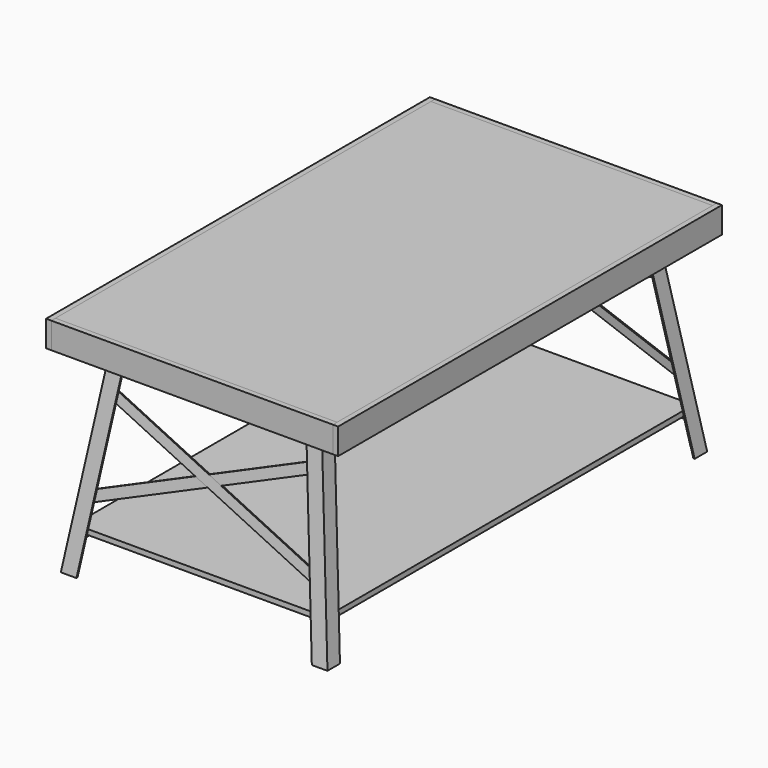
from build123d import *

# Parameters (mm, degrees)
F0_W      = 685.8
F0_H      = 1143
F1_DEPTH  = 25.4
F2_W      = 685.8
F2_H      = 12.7
F3_DEPTH  = 63.5
F4_DEPTH  = 63.5
F7_W      = 685.8
F7_H      = 63.5
F8_DEPTH  = 12.7
F13_W     = 609.6
F13_H     = 50.8
F14_DEPTH = 3.175
F18_DEPTH = 3.175
F21_W     = 34.925
F21_H     = 34.925
F22_DEPTH = 3.175
F25_W     = 611.4661372068
F25_H     = 1118.335616345
F26_DEPTH = 12.7


# Not quite as in the source:
# - a feature of the source that left no trace in its solid (it failed there, or was rolled back) is left out


with BuildPart() as f1:
    # F0 (on Top) → F1 (new body)
    with BuildSketch(Plane.XY):
        Rectangle(F0_W, F0_H)
    extrude(amount=F1_DEPTH)


with BuildPart() as f3:
    # F2 (on face) → F3 (new body)
    with BuildSketch(Plane.XY.offset(25.4)):
        with Locations((0, -577.85)):
            Rectangle(F2_W, F2_H)
    extrude(amount=-F3_DEPTH)


with BuildPart() as f4:
    # F2 (on face) → F4 (new body)
    with BuildSketch(Plane.XY.offset(25.4)):
        Polygon((-342.9, -584.2), (-342.9, -571.5), (-342.9, 571.5), (-342.9, 584.2), (-355.6, 584.2), (-355.6, -584.2), align=None)
    extrude(amount=-F4_DEPTH)


with BuildPart() as f5_1:
    # F5: instance of F4
    add(f4.part.mirror(Plane.YZ))


with BuildPart() as f6_1:
    # F6: instance of F3
    add(f3.part.mirror(Plane.XZ))


with BuildPart() as f8:
    # F7 (on face) → F8 (new body)
    with BuildSketch(Plane(origin=(0, 0, 0), x_dir=(1, 0, 0), z_dir=(0, 0, -1))):
        with Locations((0, 488.95)):
            Rectangle(F7_W, F7_H)
    extrude(amount=F8_DEPTH)


with BuildPart() as f8b:
    # F7 (on face) → F8, piece 2 (new body)
    with BuildSketch(Plane(origin=(0, 0, 0), x_dir=(1, 0, 0), z_dir=(0, 0, -1))):
        Rectangle(F7_W, F7_H)
    extrude(amount=F8_DEPTH)


with BuildPart() as f12:
    # F12: sweep along a path in F11
    with BuildLine(Plane(origin=(0, -496.4101735589, 69.7659001467), x_dir=(1, 0, 0), z_dir=(0, -0.9902680687, 0.139173101))) as f12_path:
        Line((-254, -83.2763397607), (-324.6999352877, -586.3325186814))
    # F9 (on face) → F12 (sweep)
    with BuildSketch(Plane(origin=(0, 0, -12.7), x_dir=(1, 0, 0), z_dir=(0, 0, -1))):
        Polygon((-254, 508), (-254, 469.9), (-250.825, 469.9), (-250.825, 504.825), (-215.9, 504.825), (-215.9, 508), align=None)
    sweep(path=f12_path.line)

    # F13 (on face) → F14 (join)
    with BuildSketch(Plane(origin=(0, 0, -12.7), x_dir=(1, 0, 0), z_dir=(0, 0, -1))):
        with Locations((0, 488.95)):
            Rectangle(F13_W, F13_H)
    extrude(amount=F14_DEPTH)

    # F16: F12 across plane


with BuildPart() as f12_1:
    add(f12.part)
    add(f12.part.mirror(Plane.YZ))


with BuildPart() as f18:
    # F17 (on face) → F18 (new body)
    with BuildSketch(Plane(origin=(0, -493.2966706166, 69.3283258444), x_dir=(-1, 0, 0), z_dir=(0, 0.9902680687, -0.139173101))):
        Polygon((297.1001110228, -412.0989890367), (-263.6480910569, -174.0754990191), (-267.1830878213, -199.2283079651), (301.0836328718, -440.4432197893), align=None)
    extrude(amount=F18_DEPTH)


with BuildPart() as f19_1:
    # F19: instance of F18
    add(f18.part.mirror(Plane.YZ))


with BuildPart() as f22:
    # F21 (on offset) → F22 (new body)
    with BuildSketch(Plane(origin=(0, 0, -421.9604707683), x_dir=(1, 0, 0), z_dir=(0, 0, -1))):
        with Locations((291.4455686034, 544.8803081725)):
            Rectangle(F21_W, F21_H)
    extrude(amount=F22_DEPTH)


with BuildPart() as f23_1:
    # F23: instance of F22
    add(f22.part.mirror(Plane.YZ))


with BuildPart() as f24_1:
    # F24: instance of F8
    add(f8.part.mirror(Plane.XZ))


with BuildPart() as f24_2:
    # F24: instance of F12
    add(f12_1.part.mirror(Plane.XZ))


with BuildPart() as f24_3:
    # F24: instance of F19_1
    add(f19_1.part.mirror(Plane.XZ))


with BuildPart() as f24_4:
    # F24: instance of F18
    add(f18.part.mirror(Plane.XZ))


with BuildPart() as f24_5:
    # F24: instance of F23_1
    add(f23_1.part.mirror(Plane.XZ))


with BuildPart() as f24_6:
    # F24: instance of F22
    add(f22.part.mirror(Plane.XZ))


with BuildPart() as f26:
    # F25 (on face) → F26 (new body)
    with BuildSketch(Plane.XY.offset(-421.9604707683)):
        Rectangle(F25_W, F25_H)
    extrude(amount=F26_DEPTH)


solid = Compound([f1.part, f3.part, f4.part, f5_1.part, f6_1.part, f8.part, f8b.part, f12_1.part, f18.part, f19_1.part, f22.part, f23_1.part, f24_1.part, f24_2.part, f24_3.part, f24_4.part, f24_5.part, f24_6.part, f26.part])
